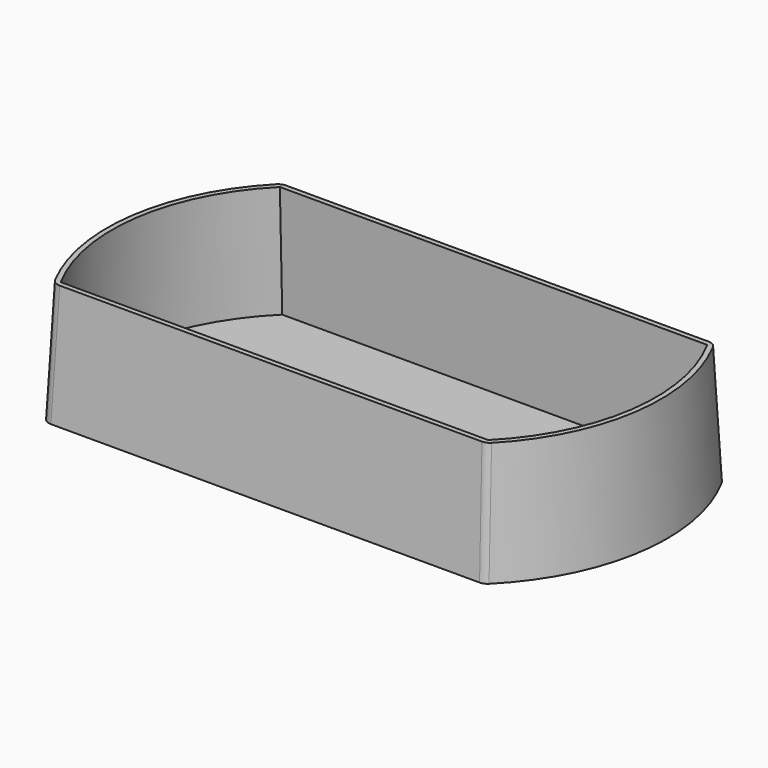
from build123d import *

# Parameters (mm, degrees)
F1_DEPTH               = 60
DRAFT_F1_DRAFTED_ANGLE = -3
F2_T                   = -2.5
F3_R                   = 5


# Not quite as in the source:
# - an extrude with a draft is written as a straight extrude whose walls are then drafted


with BuildPart() as f1:
    # F0 (on Top) → F1 (new body)
    with BuildSketch(Plane.XY):
        with BuildLine():
            Line((117.118632605, 42.652064257), (-97.881367395, 42.652064257))
            ThreePointArc((-97.881367395, 42.652064257), (-126.8175686365, -14.7972991315), (-114.7763384734, -77.985445743))
            Line((-114.7763384734, -77.985445743), (100.2236615266, -77.985445743))
            ThreePointArc((100.2236615266, -77.985445743), (129.1598627681, -20.5360823545), (117.118632605, 42.652064257))
        make_face()
    extrude(amount=-F1_DEPTH)

    # draft_F1_drafted
    draft_f1_drafted_walls = [f1.faces().sort_by_distance(p)[0] for p in [
        (-7.2763384734, -77.985445743, -40),
        (129.1598627681, -20.5360823545, -40),
        (9.618632605, 42.652064257, -40),
        (-126.8175686365, -14.7972991315, -40),
    ]]
    draft(draft_f1_drafted_walls, neutral_plane=Plane(origin=(0, 0, 0), x_dir=(1, 0, 0), z_dir=(0, 0, -1)), angle=DRAFT_F1_DRAFTED_ANGLE)

    # F2
    f2_openings = [f1.faces().sort_by_distance(p)[0] for p in [
        (1.171147, -17.666691, 0),
    ]]
    offset(amount=F2_T, openings=f2_openings, kind=Kind.INTERSECTION)

    # F3
    f3_edges = [f1.edges().sort_by_distance(p)[0] for p in [
        (-115.682866, -79.549572, -29.8453),
        (100.861164, -79.550594, -29.864812),
        (118.025161, 44.21619, -29.8453),
        (-98.51887, 44.217213, -29.864812),
    ]]
    fillet(f3_edges, radius=F3_R)


solid = f1.part
